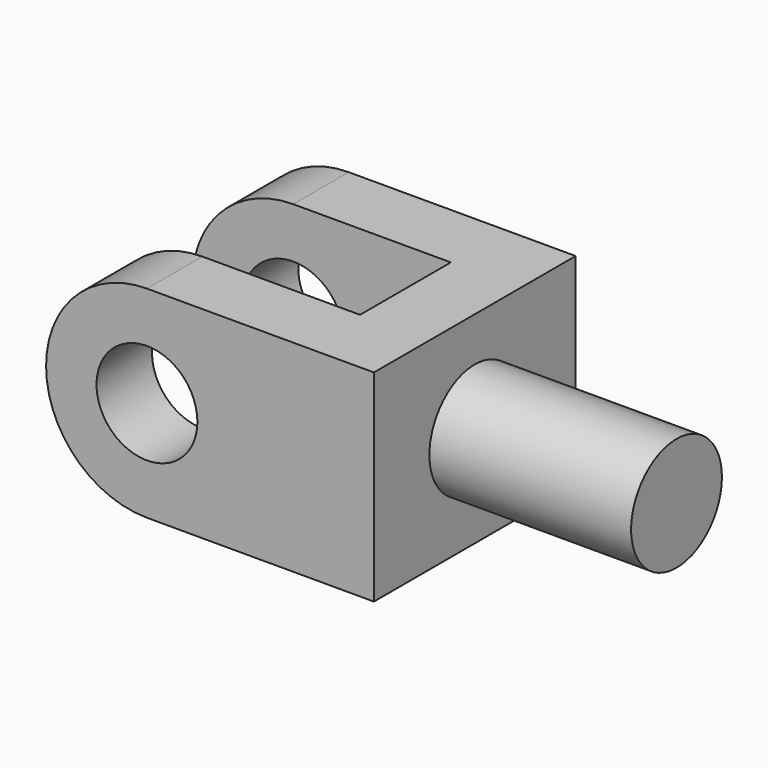
from build123d import *

# Parameters (mm, degrees)
F0_W     = 52
F0_H     = 32
F1_DEPTH = 40
F2_R     = 15.99999
F3_R     = 8
F4_DEPTH = 40.001
F5_W     = 26.99999
F5_H     = 18
F5_W_2   = 25.00001
F6_DEPTH = 32.001
F7_R     = 9
F8_DEPTH = 32


# Not quite as in the source:
# - a fillet or chamfer is up to 0.001 mm smaller than in the source, because OpenCascade refuses the exact size


with BuildPart() as f1:
    # F0 (on Front) → F1 (new body)
    with BuildSketch(Plane.XZ):
        with Locations((6.3565019518, 4.5450745088)):
            Rectangle(F0_W, F0_H)
    extrude(amount=F1_DEPTH)

    # F2 (radius 16 in the source; OpenCascade refuses exactly that, so slightly less here)
    f2_edges = [f1.edges().sort_by_distance(p)[0] for p in [
        (-19.643498, -20, 20.545075),
        (-19.643498, -20, -11.454925),
    ]]
    fillet(f2_edges, radius=F2_R)

    # F3 (on face) → F4 (cut, through all)
    with BuildSketch(Plane.XZ.offset(40)):
        with Locations((-3.6434980482, 4.5450745088)):
            Circle(F3_R)
    extrude(amount=-F4_DEPTH, mode=Mode.SUBTRACT)

    # F5 (on face) → F6 (cut, through all)
    with BuildSketch(Plane.XY.offset(20.5450745088)):
        with Locations((-17.1435030482, -20)):
            Rectangle(F5_W, F5_H)
        with Locations((8.8564969518, -20)):
            Rectangle(F5_W_2, F5_H)
    extrude(amount=-F6_DEPTH, mode=Mode.SUBTRACT)

    # F7 (on face) → F8 (join)
    with BuildSketch(Plane.YZ.offset(32.3565019518)):
        with Locations((-20, 4.5450745088)):
            Circle(F7_R)
    extrude(amount=F8_DEPTH)


solid = f1.part
